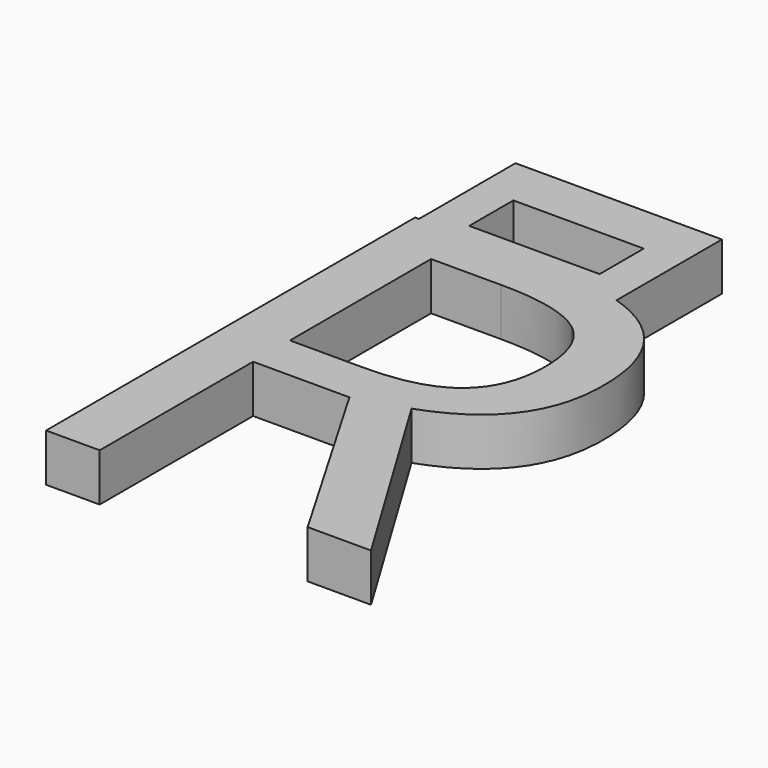
from build123d import *

# Parameters (mm, degrees)
F0_W     = 4.318
F0_H     = 1.4593527386
F1_DEPTH = 2


with BuildPart() as f1:
    # F0 (on Top) → F1 (new body)
    with BuildSketch(Plane.XY):
        with Locations((4.9730502656, -0.8943877724)):
            Rectangle(F0_W, F0_H)
        with BuildLine():
            Line((7.1320502656, -1.6240641417), (2.8140502656, -1.6240641417))
            Line((2.8140502656, -1.6240641417), (2.8140502656, -0.1647114031))
            Line((2.8140502656, -0.1647114031), (2.6522759268, -0.1647114031))
            Line((2.6522759268, -0.1647114031), (2.6522759268, -19.4612857813))
            Line((2.6522759268, -19.4612857813), (4.8948850305, -19.4612857813))
            Line((4.8948850305, -19.4612857813), (4.8948850305, -11.436884092))
            Line((4.8948850305, -11.436884092), (8.9239793524, -11.436884092))
            Line((8.9239793524, -11.436884092), (13.5950258095, -19.4612857813))
            Line((13.5950258095, -19.4612857813), (16.2473017363, -19.4612857813))
            Line((16.2473017363, -19.4612857813), (11.0061004223, -10.7907085875))
            add(Edge.make_bspline(
                [(14.8873768184, -5.6170811825), (14.8873768184, -9.4434537776), (11.0061004223, -10.7907085875)],
                knots=[0, 0, 0, 1, 1, 1], degree=2))
            add(Edge.make_bspline(
                [(13.1916940404, -1.524636321), (14.8873768184, -2.8845612389), (14.8873768184, -5.6170811825)],
                knots=[0, 0, 0, 1, 1, 1], degree=2))
            add(Edge.make_bspline(
                [(11.4500502656, -0.6254353556), (12.4829894147, -0.9562605066), (13.1916940404, -1.524636321)],
                knots=[0.5820535333, 0.5820535333, 0.5820535333, 1, 1, 1], degree=2))
            Line((11.4500502656, -0.6254353556), (11.4500502656, -1.6240641417))
            Line((11.4500502656, -1.6240641417), (7.1320502656, -1.6240641417))
        make_face()
        with BuildLine():
            Line((7.9737212576, -9.5110276865), (4.8948850305, -9.5110276865))
            Line((4.8948850305, -9.5110276865), (4.8948850305, -2.1328015016))
            Line((4.8948850305, -2.1328015016), (7.8132332238, -2.1328015016))
            add(Edge.make_bspline(
                [(11.436884092, -2.9774753637), (10.3092444862, -2.1328015016), (7.8132332238, -2.1328015016)],
                knots=[0, 0, 0, 1, 1, 1], degree=2))
            add(Edge.make_bspline(
                [(12.5645236978, -5.7353355232), (12.5645236978, -3.8221492257), (11.436884092, -2.9774753637)],
                knots=[0, 0, 0, 1, 1, 1], degree=2))
            add(Edge.make_bspline(
                [(11.4558892539, -8.5671046457), (12.5645236978, -7.6231816049), (12.5645236978, -5.7353355232)],
                knots=[0, 0, 0, 1, 1, 1], degree=2))
            add(Edge.make_bspline(
                [(7.9737212576, -9.5110276865), (10.3472548099, -9.5110276865), (11.4558892539, -8.5671046457)],
                knots=[0, 0, 0, 1, 1, 1], degree=2))
        make_face(mode=Mode.SUBTRACT)
        with BuildLine():
            Line((7.1320502656, -0.1647114031), (7.1320502656, -1.6240641417))
            Line((7.1320502656, -1.6240641417), (11.4500502656, -1.6240641417))
            Line((11.4500502656, -1.6240641417), (11.4500502656, -0.6254353556))
            add(Edge.make_bspline(
                [(7.9441576725, -0.1647114031), (10.0115266043, -0.1647114031), (11.4500502656, -0.6254353556)],
                knots=[0, 0, 0, 0.5820535333, 0.5820535333, 0.5820535333], degree=2))
            Line((7.9441576725, -0.1647114031), (7.1320502656, -0.1647114031))
        make_face()
        Polygon((2.8140502656, 4.8854069319), (2.8140502656, -0.1647114031), (7.1320502656, -0.1647114031), (7.1320502656, 0.4763843317), (4.4037376737, 0.4763843317), (4.4037376737, 2.7849584585), (7.1320502656, 2.7849584585), (7.1320502656, 4.8854069319), align=None)
        with BuildLine():
            Line((7.1320502656, 0.4763843317), (7.1320502656, -0.1647114031))
            Line((7.1320502656, -0.1647114031), (7.9441576725, -0.1647114031))
            add(Edge.make_bspline(
                [(7.9441576725, -0.1647114031), (10.0115266043, -0.1647114031), (11.4500502656, -0.6254353556)],
                knots=[0, 0, 0, 0.5820535333, 0.5820535333, 0.5820535333], degree=2))
            Line((11.4500502656, -0.6254353556), (11.4500502656, 4.8854069319))
            Line((11.4500502656, 4.8854069319), (7.1320502656, 4.8854069319))
            Line((7.1320502656, 4.8854069319), (7.1320502656, 2.7849584585))
            Line((7.1320502656, 2.7849584585), (9.8603628576, 2.7849584585))
            Line((9.8603628576, 2.7849584585), (9.8603628576, 0.4763843317))
            Line((9.8603628576, 0.4763843317), (7.1320502656, 0.4763843317))
        make_face()
    extrude(amount=F1_DEPTH)


solid = f1.part
